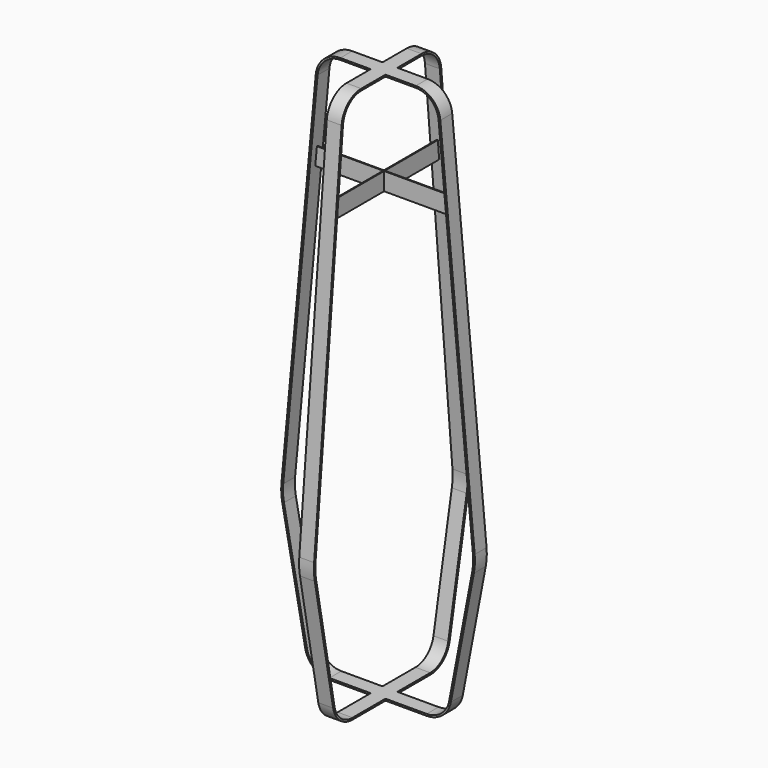
from build123d import *

# Parameters (mm, degrees)
F2_W          = 50
F2_H          = 6
F6_DEPTH      = 12
F4_W          = 3
F4_H          = 60
F8_DEPTH      = 230.3205006971
F8_DEPTH_BACK = 230.3205006971
F9_COUNT      = 3
F9_ANGLE      = 180


with BuildPart() as f3:
    # F3: sweep along a path in F1
    with BuildLine(Plane.XZ) as f3_path:
        Line((0, 0), (163.7688020474, 0))
        ThreePointArc((163.7688020474, 0), (214.7853281283, 18.3776496177), (242.3627581835, 65.0671483341))
        Line((242.3627581835, 65.0671483341), (319.737347904, 472.3018310739))
        ThreePointArc((319.737347904, 472.3018310739), (323.0248161759, 500.0943200705), (322.4005923749, 528.0736023507))
        Line((322.4005923749, 528.0736023507), (206.7244576996, 1777.3758568449))
        ThreePointArc((206.7244576996, 1777.3758568449), (180.9629377368, 1829.1188148883), (127.0652037751, 1850))
        Line((127.0652037751, 1850), (0, 1850))
    # F2 (on Right) → F3 (sweep)
    with BuildSketch(Plane.YZ):
        Rectangle(F2_W, F2_H)
    sweep(path=f3_path.line)

    # F7: F3 across plane


with BuildPart() as f6:
    # F5 (on Right) → F6 (new body)
    with BuildSketch(Plane.YZ):
        with BuildLine():
            Line((-1.5, 1490), (1.5, 1490))
            Line((1.5, 1490), (1.5, 1504))
            ThreePointArc((1.5, 1504), (3.5502525317, 1508.9497474683), (8.5, 1511))
            Line((8.5, 1511), (24.5, 1511))
            ThreePointArc((24.5, 1511), (31.5710678119, 1513.9289321881), (34.5, 1521))
            Line((34.5, 1521), (34.5, 1527))
            Line((34.5, 1527), (31.5, 1527))
            Line((31.5, 1527), (31.5, 1521))
            ThreePointArc((31.5, 1521), (29.4497474683, 1516.0502525317), (24.5, 1514))
            Line((24.5, 1514), (8.5, 1514))
            ThreePointArc((8.5, 1514), (1.4289321881, 1511.0710678119), (-1.5, 1504))
            Line((-1.5, 1504), (-1.5, 1490))
        make_face()
    extrude(amount=F6_DEPTH)


with BuildPart() as f3_1:
    add(f3.part)
    add(f3.part.mirror(Plane.YZ))

    # F4 (on Right) → F8 (join, two sides)
    with BuildSketch(Plane.YZ) as f8_sk:
        with Locations((0, 1520)):
            Rectangle(F4_W, F4_H)
    extrude(amount=F8_DEPTH)
    extrude(f8_sk.sketch, amount=-F8_DEPTH_BACK)

    # F9: F3 ×3 about axis
    f9_axis = Axis((0, 0, 925), (0, 0, -1))


with BuildPart() as f3_2:
    add(f3_1.part)
    for i in range(1, F9_COUNT):
        add(f3_1.part.rotate(f9_axis, i * F9_ANGLE / (F9_COUNT - 1)))


solid = Compound([f6.part, f3_2.part])
